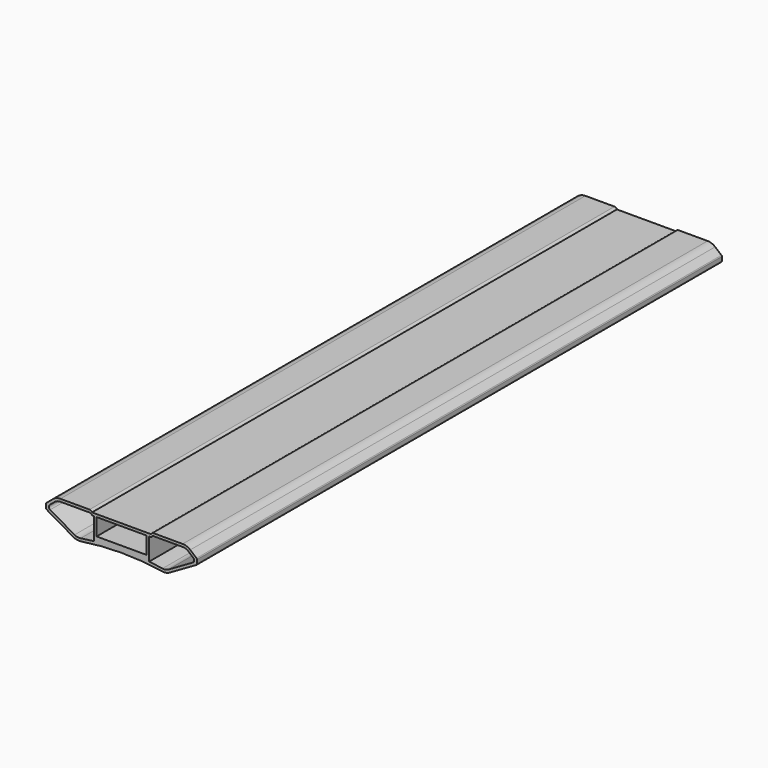
from build123d import *

# Parameters (mm, degrees)
F1_DEPTH    = 250
F2_W        = 38
F2_H        = 13
F3_DEPTH    = 250
F4_T1_DEPTH = 509.3674969976
F5_R        = 9
F6_R        = 1
F8_DEPTH    = 250


# Not quite as in the source:
# - a fillet or chamfer that OpenCascade refuses, or shapes differently, is made with other operations: its cross-section is extruded or revolved along the edge and cut away or added


with BuildPart() as f1:
    # F0 (on Front) → F1 (new body, symmetric)
    with BuildSketch(Plane.XZ):
        with BuildLine():
            Line((22.5, 0), (0, 0))
            Line((0, 0), (-22.5, 0))
            Line((-22.5, 0), (-22.5, 1.3))
            Line((-22.5, 1.3), (-49.8395555688, 1.3))
            Line((-49.8395555688, 1.3), (-57.5, -5.1278760969))
            Line((-57.5, -5.1278760969), (-57.5, -9.1278760969))
            Line((-57.5, -9.1278760969), (-33.9923918332, -22.7))
            ThreePointArc((-33.9923918332, -22.7), (0, -19.7901248096), (33.9923918332, -22.7))
            Line((33.9923918332, -22.7), (57.5, -9.1278760969))
            Line((57.5, -9.1278760969), (57.5, -5.1278760969))
            Line((57.5, -5.1278760969), (49.8395555688, 1.3))
            Line((49.8395555688, 1.3), (22.5, 1.3))
            Line((22.5, 1.3), (22.5, 0))
        make_face()
    extrude(amount=F1_DEPTH, both=True)

    # F2 (on Front) → F3 (cut, symmetric)
    with BuildSketch(Plane.XZ):
        with Locations((0, -8.5)):
            Rectangle(F2_W, F2_H)
    extrude(amount=F3_DEPTH, both=True, mode=Mode.SUBTRACT)

    # F4: fillet of radius 2 on 2 edges, made by hand

    # F4_s2 → F4_t1 (cut)
    with BuildSketch(Plane.XZ.offset(-254.6837484988)):
        with BuildLine():
            ThreePointArc((-24.3734993995, 1.3), (-23.2333239744, 0.9431676725), (-22.5, 0))
            Line((-22.5, 0), (-22.5, 1.3))
            Line((-22.5, 1.3), (-24.3734993995, 1.3))
        make_face()
        with BuildLine():
            ThreePointArc((24.3734993995, 1.3), (23.2333239744, 0.9431676725), (22.5, 0))
            Line((22.5, 0), (22.5, 1.3))
            Line((22.5, 1.3), (24.3734993995, 1.3))
        make_face()
    extrude(amount=F4_T1_DEPTH, mode=Mode.SUBTRACT)

    # F5
    f5_edges = [f1.edges().sort_by_distance(p)[0] for p in [
        (-49.839556, 0, 1.3),
        (49.839556, 0, 1.3),
        (33.992392, 0, -22.7),
        (-33.992392, 0, -22.7),
    ]]
    fillet(f5_edges, radius=F5_R)

    # F6
    f6_edges = [f1.edges().sort_by_distance(p)[0] for p in [
        (-57.5, 0, -5.127876),
        (57.5, 0, -5.127876),
        (57.5, 0, -9.127876),
        (-57.5, 0, -9.127876),
    ]]
    fillet(f6_edges, radius=F6_R)

    # F7 (on Front) → F8 (cut, symmetric)
    with BuildSketch(Plane.XZ):
        with BuildLine():
            ThreePointArc((-35.7777574473, -19.3598176053), (-33.5603570371, -20.1791322254), (-31.1966842313, -20.2136560239))
            ThreePointArc((-31.1966842313, -20.2136560239), (-26.106800057, -19.4842711987), (-21, -18.8846744107))
            Line((-21, -18.8846744107), (-21, -2))
            Line((-21, -2), (-22.5, -2))
            ThreePointArc((-22.5, -2), (-23.2333239744, -1.0568323275), (-24.3734993995, -0.7))
            Line((-24.3734993995, -0.7), (-46.5638234604, -0.7))
            ThreePointArc((-46.5638234604, -0.7), (-48.9579644637, -1.1221516545), (-51.0633367282, -2.3376888982))
            Line((-51.0633367282, -2.3376888982), (-54.6622869129, -5.3575666708))
            ThreePointArc((-54.6622869129, -5.3575666708), (-55.3691010897, -7.0639670425), (-54.3767116936, -8.6217063646))
            Line((-54.3767116936, -8.6217063646), (-35.7777574473, -19.3598176053))
        make_face()
        with BuildLine():
            Line((22.5, -2), (21, -2))
            Line((21, -2), (21, -18.8846744107))
            ThreePointArc((21, -18.8846744107), (26.106800057, -19.4842711987), (31.1966842313, -20.2136560239))
            ThreePointArc((31.1966842313, -20.2136560239), (33.5603570371, -20.1791322254), (35.7777574473, -19.3598176053))
            Line((35.7777574473, -19.3598176053), (54.3767116936, -8.6217063646))
            ThreePointArc((54.3767116936, -8.6217063646), (55.3691010897, -7.0639670425), (54.6622869129, -5.3575666708))
            Line((54.6622869129, -5.3575666708), (51.0633367282, -2.3376888982))
            ThreePointArc((51.0633367282, -2.3376888982), (48.9579644637, -1.1221516545), (46.5638234604, -0.7))
            Line((46.5638234604, -0.7), (24.3734993995, -0.7))
            ThreePointArc((24.3734993995, -0.7), (23.2333239744, -1.0568323275), (22.5, -2))
        make_face()
    extrude(amount=F8_DEPTH, both=True, mode=Mode.SUBTRACT)


solid = f1.part
